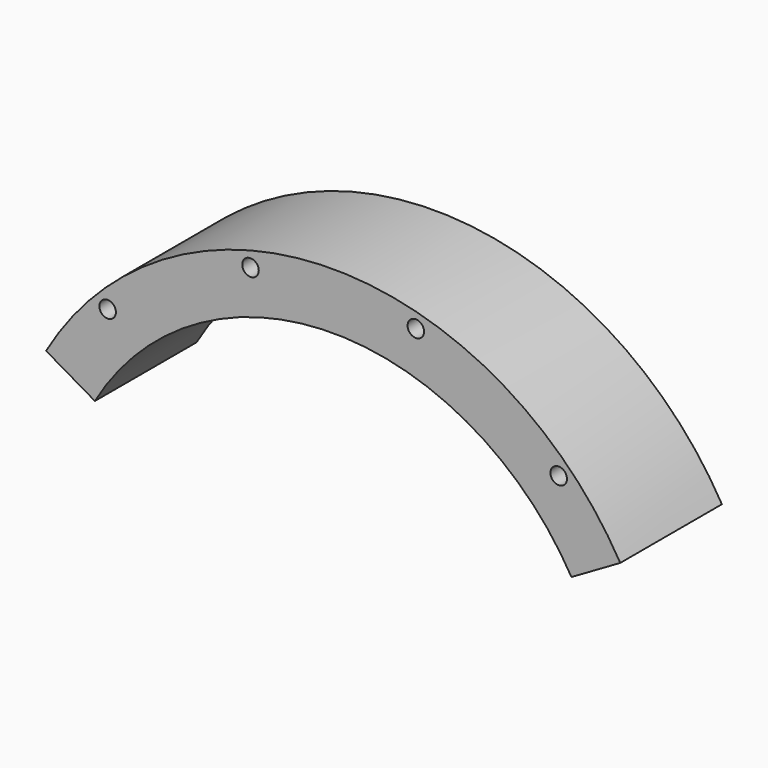
from build123d import *

# Parameters (mm, degrees)
F0_R     = 0.325
F1_DEPTH = 5


# Not quite as in the source:
# - ends of sketch curves that miss each other by under 0.0002 mm in the source are joined


with BuildPart() as f1:
    # F0 (on Front) → F1 (new body)
    with BuildSketch(Plane.XZ):
        with BuildLine():
            Line((-11.295323, -2.696106), (-9.375, -3.81))
            ThreePointArc((-9.375, -3.81), (0, 1.590001), (9.3750005059, -3.8099997066))
            Line((9.3750005059, -3.8099997066), (11.295323, -2.696106))
            ThreePointArc((11.295323, -2.696106), (0, 3.810001), (-11.295323, -2.696106))
        make_face()
        with Locations((-8.873374, -0.467984)):
            Circle(F0_R, mode=Mode.SUBTRACT)
        with Locations((8.873374, -0.467984)):
            Circle(F0_R, mode=Mode.SUBTRACT)
        with Locations((-3.2525, 2.803828)):
            Circle(F0_R, mode=Mode.SUBTRACT)
        with Locations((3.2525, 2.803828)):
            Circle(F0_R, mode=Mode.SUBTRACT)
    extrude(amount=F1_DEPTH)


solid = f1.part
